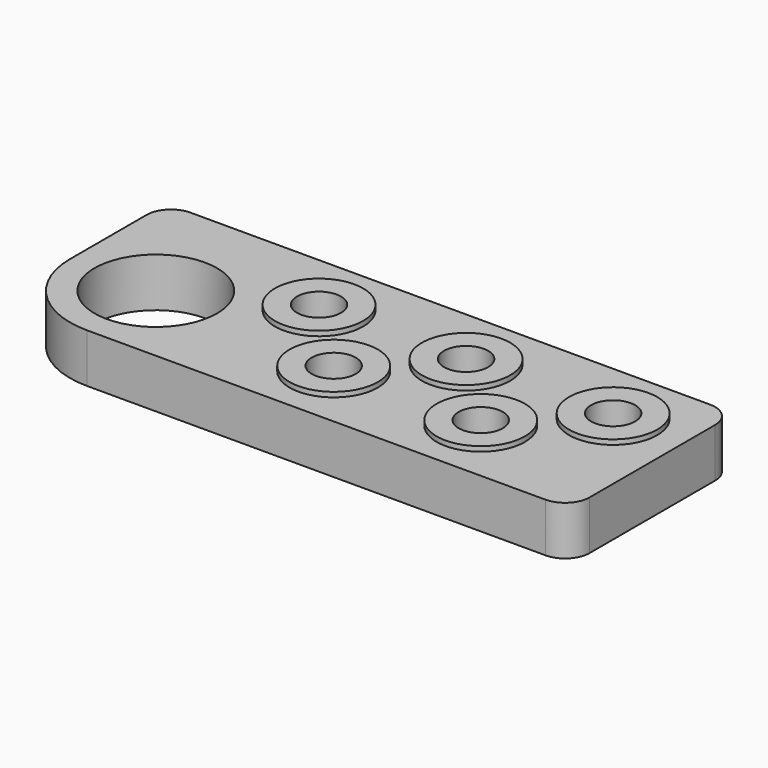
from build123d import *

# Parameters (mm, degrees)
F0_R         = 12.5
F1_DEPTH     = 10
F2_R         = 9
F2_R_2       = 4.5
F3_DEPTH     = 1
F4_DEPTH     = 9
F5_TEXT_SIZE = 5.5555555556
F6_DEPTH     = 1


# Not quite as in the source:
# - Text() gives the source's letters only with a copy of the font that has no kerning and outlines rounded to 1/6400 em; it was checked with that copy


with BuildPart() as f1:
    # F0 (on Top) → F1 (new body)
    with BuildSketch(Plane.XY):
        with BuildLine():
            ThreePointArc((0, 17.5), (5.1256313292, 5.1256313292), (17.5, 0))
            Line((17.5, 0), (111, 0))
            ThreePointArc((111, 0), (114.5355339059, 1.4644660941), (116, 5))
            Line((116, 5), (116, 37))
            ThreePointArc((116, 37), (114.5355339059, 40.5355339059), (111, 42))
            Line((111, 42), (5, 42))
            ThreePointArc((5, 42), (1.4644660941, 40.5355339059), (0, 37))
            Line((0, 37), (0, 17.5))
        make_face()
        with Locations((17.5, 17.5)):
            Circle(F0_R, mode=Mode.SUBTRACT)
    extrude(amount=F1_DEPTH)

    # F2 (on face) → F3 (join)
    with BuildSketch(Plane.XY.offset(10)):
        with Locations((42, 28.5)):
            Circle(F2_R)
        with Locations((42, 28.5)):
            Circle(F2_R_2, mode=Mode.SUBTRACT)
        with Locations((57, 13.5)):
            Circle(F2_R)
        with Locations((57, 13.5)):
            Circle(F2_R_2, mode=Mode.SUBTRACT)
        with Locations((72, 28.5)):
            Circle(F2_R)
        with Locations((72, 28.5)):
            Circle(F2_R_2, mode=Mode.SUBTRACT)
        with Locations((87, 13.5)):
            Circle(F2_R)
        with Locations((87, 13.5)):
            Circle(F2_R_2, mode=Mode.SUBTRACT)
        with Locations((102, 28.5)):
            Circle(F2_R)
        with Locations((102, 28.5)):
            Circle(F2_R_2, mode=Mode.SUBTRACT)
    extrude(amount=F3_DEPTH)

    # F4 (cut): faces of the model
    f4_faces = [f1.faces().sort_by_distance(p)[0] for p in [
        (42, 28.5, 10),
        (57, 13.5, 10),
        (72, 28.5, 10),
        (87, 13.5, 10),
        (102, 28.5, 10),
    ]]
    extrude(f4_faces, amount=-F4_DEPTH, mode=Mode.SUBTRACT)

    # F5 (on face) → F6 (cut)
    with BuildSketch(Plane(origin=(0, 0, 0), x_dir=(1, 0, 0), z_dir=(0, 0, -1))):
        with Locations((30, -9)):
            Text('963', F5_TEXT_SIZE, font='Open Sans', text_align=(TextAlign.LEFT, TextAlign.BOTTOM))
    extrude(amount=-F6_DEPTH, mode=Mode.SUBTRACT)


solid = f1.part
